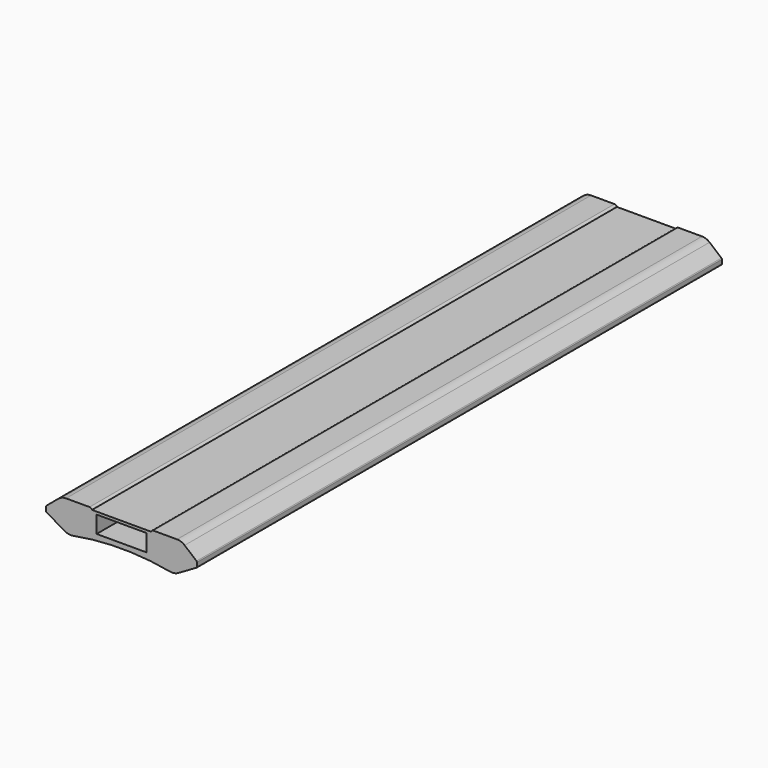
from build123d import *

# Parameters (mm, degrees)
F1_DEPTH    = 250
F2_W        = 38
F2_H        = 13
F3_DEPTH    = 250
F4_T1_DEPTH = 509.3674969976
F5_R        = 9
F6_R        = 1


# Not quite as in the source:
# - a fillet or chamfer that OpenCascade refuses, or shapes differently, is made with other operations: its cross-section is extruded or revolved along the edge and cut away or added


with BuildPart() as f1:
    # F0 (on Front) → F1 (new body, symmetric)
    with BuildSketch(Plane.XZ):
        with BuildLine():
            Line((22.5, 23.1507345177), (0, 23.1507345177))
            Line((0, 23.1507345177), (-22.5, 23.1507345177))
            Line((-22.5, 23.1507345177), (-22.5, 24.4507345177))
            Line((-22.5, 24.4507345177), (-45.5824640741, 24.4507345177))
            Line((-45.5824640741, 24.4507345177), (-57.5, 14.4507345177))
            Line((-57.5, 14.4507345177), (-57.5, 10.4507345177))
            Line((-57.5, 10.4507345177), (-40.1794919243, 0.4507345177))
            ThreePointArc((-40.1794919243, 0.4507345177), (0, 4.5282793762), (40.1794919243, 0.4507345177))
            Line((40.1794919243, 0.4507345177), (57.5, 10.4507345177))
            Line((57.5, 10.4507345177), (57.5, 14.4507345177))
            Line((57.5, 14.4507345177), (45.5824640741, 24.4507345177))
            Line((45.5824640741, 24.4507345177), (22.5, 24.4507345177))
            Line((22.5, 24.4507345177), (22.5, 23.1507345177))
        make_face()
    extrude(amount=F1_DEPTH, both=True)

    # F2 (on Front) → F3 (cut, symmetric)
    with BuildSketch(Plane.XZ):
        with Locations((0, 14.6507345177)):
            Rectangle(F2_W, F2_H)
    extrude(amount=F3_DEPTH, both=True, mode=Mode.SUBTRACT)

    # F4: fillet of radius 2 on 2 edges, made by hand

    # F4_s2 → F4_t1 (cut)
    with BuildSketch(Plane.XZ.offset(-254.6837484988)):
        with BuildLine():
            ThreePointArc((-24.3734993995, 24.4507345177), (-23.2333239744, 24.0939021903), (-22.5, 23.1507345177))
            Line((-22.5, 23.1507345177), (-22.5, 24.4507345177))
            Line((-22.5, 24.4507345177), (-24.3734993995, 24.4507345177))
        make_face()
        with BuildLine():
            ThreePointArc((24.3734993995, 24.4507345177), (23.2333239744, 24.0939021903), (22.5, 23.1507345177))
            Line((22.5, 23.1507345177), (22.5, 24.4507345177))
            Line((22.5, 24.4507345177), (24.3734993995, 24.4507345177))
        make_face()
    extrude(amount=F4_T1_DEPTH, mode=Mode.SUBTRACT)

    # F5
    f5_edges = [f1.edges().sort_by_distance(p)[0] for p in [
        (45.582464, 0, 24.450735),
        (40.179492, 0, 0.450735),
        (-45.582464, 0, 24.450735),
        (-40.179492, 0, 0.450735),
    ]]
    fillet(f5_edges, radius=F5_R)

    # F6
    f6_edges = [f1.edges().sort_by_distance(p)[0] for p in [
        (57.5, 0, 14.450735),
        (57.5, 0, 10.450735),
        (-57.5, 0, 14.450735),
        (-57.5, 0, 10.450735),
    ]]
    fillet(f6_edges, radius=F6_R)


solid = f1.part
